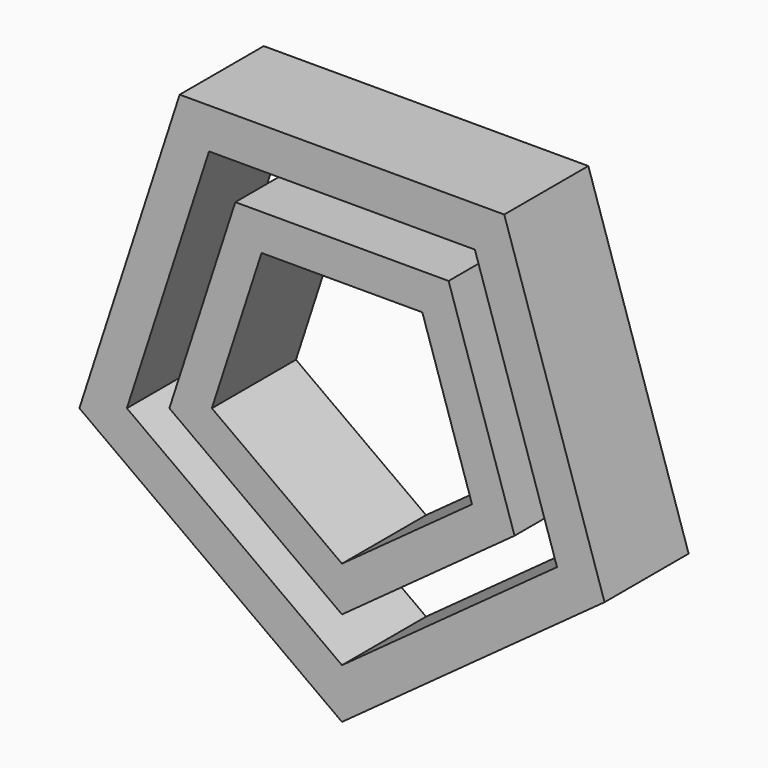
from build123d import *

# Parameters (mm, degrees)
F1_DEPTH = 457.2
F2_DEPTH = 457.2
F3_DEPTH = 457.2


with BuildPart() as f1:
    # F0 (on Front) → F1 (new body)
    with BuildSketch(Plane.XZ):
        Polygon((-1142.0303102433, -371.068141493), (0, -1200.8017301559), (1142.0303102433, -371.068141493), (705.813547913, 971.469006571), (-705.813547913, 971.469006571), align=None)
        Polygon((935.4130086182, -303.9341106125), (0, -983.5514426231), (-935.4130086182, -303.9341106125), (-578.1170328449, 795.7098319241), (578.1170328449, 795.7098319241), align=None, mode=Mode.SUBTRACT)
    extrude(amount=F1_DEPTH)

    # F0 (on Front) → F3 (cut)
    with BuildSketch(Plane.XZ):
        Polygon((-407.9753176564, -132.5592162834), (0, -428.9706349373), (407.9753176564, -132.5592162834), (252.1426128827, 347.0445337521), (-252.1426128827, 347.0445337521), align=None)
        Polygon((281.7509045029, -91.5464183044), (0, -296.2504327297), (-281.7509045029, -91.5464183044), (-174.1316353438, 239.6716346693), (174.1316353438, 239.6716346693), align=None, mode=Mode.SUBTRACT)
    extrude(amount=F3_DEPTH, mode=Mode.SUBTRACT)


with BuildPart() as f2:
    # F0 (on Front) → F2 (new body)
    with BuildSketch(Plane.XZ):
        Polygon((-750.5844107294, -243.8796587313), (0, -789.2111539841), (750.5844107294, -243.8796587313), (463.8866772566, 638.4852357234), (-463.8866772566, 638.4852357234), align=None)
        Polygon((565.7558128405, -183.8252068501), (0, -594.870865345), (-565.7558128405, -183.8252068501), (-349.6563216683, 481.2606395226), (349.6563216683, 481.2606395226), align=None, mode=Mode.SUBTRACT)
    extrude(amount=F2_DEPTH)


solid = Compound([f1.part, f2.part])
